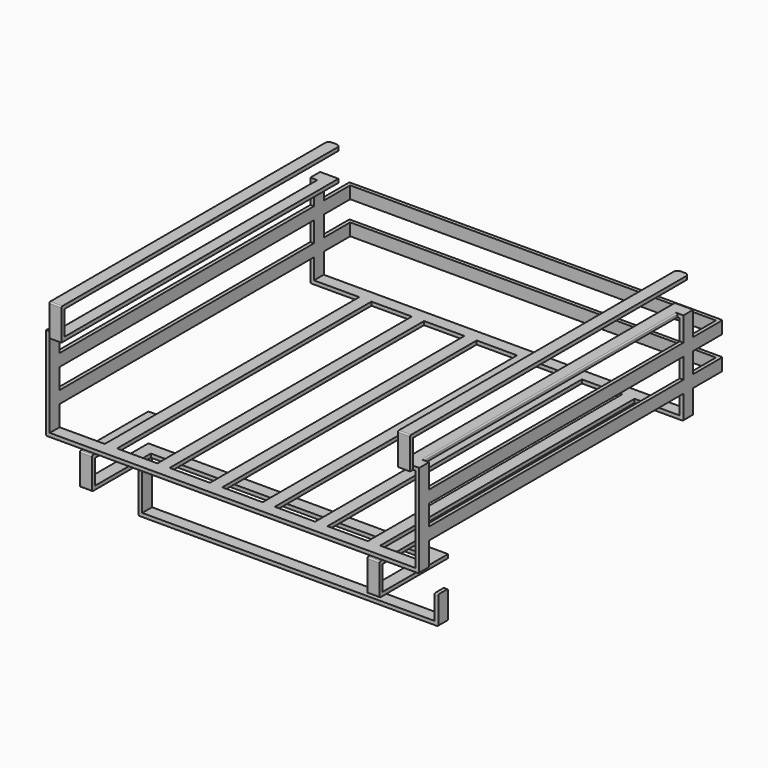
from build123d import *

# Parameters (mm, degrees)
F0_W           = 10
F0_H           = 260
F1_DEPTH       = 3
F2_W           = 3
F2_H           = 10
F3_DEPTH       = 70
F4_W           = 2
F4_H           = 10
F4_W_2         = 3
F4_W_3         = 10
F4_H_2         = 3
F4_W_4         = 5
F5_DEPTH       = 3
F6_W           = 10
F6_H           = 3
F7_DEPTH       = 20
F8_W           = 10
F8_H           = 282
F8_H_2         = 285
F8_H_3         = 3
F9_DEPTH       = 3
F10_W          = 3
F10_H          = 10
F11_DEPTH      = 30
F11_DEPTH_BACK = 270
F12_W          = 3
F12_H          = 10
F13_DEPTH      = 299
F14_R          = 1
F15_R          = 3
F16_W          = 10
F16_H          = 70
F17_DEPTH      = 3
F18_W          = 10
F18_H          = 3
F19_DEPTH      = 20
F20_W          = 10
F20_H          = 70
F21_DEPTH      = 3
F20_H_2        = 67
F20_H_3        = 3
F22_W          = 10
F22_H          = 3
F23_DEPTH      = 225
F24_W          = 3
F24_H          = 10
F25_DEPTH      = 45
F26_W          = 10
F26_H          = 3
F27_DEPTH      = 242
F28_W          = 3
F28_H          = 10
F29_DEPTH      = 20
F30_R          = 1
F32_DEPTH      = 1


with BuildPart() as f1:
    # F0 (on Top) → F1 (new body)
    with BuildSketch(Plane.XY):
        Polygon((135.7191348076, 185.6500792865), (-169.2808651924, 185.6500792865), (-169.2808651924, 175.6500792865), (-129.2808651924, 175.6500792865), (-119.2808651924, 175.6500792865), (-86.2808651924, 175.6500792865), (-76.2808651924, 175.6500792865), (-43.2808651924, 175.6500792865), (-33.2808651924, 175.6500792865), (-0.2808651924, 175.6500792865), (9.7191348076, 175.6500792865), (42.7191348076, 175.6500792865), (52.7191348076, 175.6500792865), (85.7191348076, 175.6500792865), (95.7191348076, 175.6500792865), (135.7191348076, 175.6500792865), align=None)
        with Locations((-124.2808651924, 45.6500792865)):
            Rectangle(F0_W, F0_H)
        with Locations((-81.2808651924, 45.6500792865)):
            Rectangle(F0_W, F0_H)
        with Locations((-38.2808651924, 45.6500792865)):
            Rectangle(F0_W, F0_H)
        with Locations((4.7191348076, 45.6500792865)):
            Rectangle(F0_W, F0_H)
        with Locations((47.7191348076, 45.6500792865)):
            Rectangle(F0_W, F0_H)
        with Locations((90.7191348076, 45.6500792865)):
            Rectangle(F0_W, F0_H)
        Polygon((-129.2808651924, -84.3499207135), (-169.2808651924, -84.3499207135), (-169.2808651924, -94.3499207135), (135.7191348076, -94.3499207135), (135.7191348076, -84.3499207135), (95.7191348076, -84.3499207135), (85.7191348076, -84.3499207135), (52.7191348076, -84.3499207135), (42.7191348076, -84.3499207135), (9.7191348076, -84.3499207135), (-0.2808651924, -84.3499207135), (-33.2808651924, -84.3499207135), (-43.2808651924, -84.3499207135), (-76.2808651924, -84.3499207135), (-86.2808651924, -84.3499207135), (-119.2808651924, -84.3499207135), align=None)
    extrude(amount=F1_DEPTH)

    # F2 (on face) → F3 (join)
    with BuildSketch(Plane.XY.offset(3)):
        with Locations((-167.7808651924, 180.6500792865)):
            Rectangle(F2_W, F2_H)
        with Locations((134.2191348076, 180.6500792865)):
            Rectangle(F2_W, F2_H)
        with Locations((134.2191348076, -89.3499207135)):
            Rectangle(F2_W, F2_H)
        with Locations((-167.7808651924, -89.3499207135)):
            Rectangle(F2_W, F2_H)
    extrude(amount=F3_DEPTH)

    # F4 (on face) → F5 (join)
    with BuildSketch(Plane.XY.offset(73)):
        Polygon((-154.2808651924, 185.6500792865), (-164.2808651924, 185.6500792865), (-164.2808651924, 175.6500792865), (-164.2808651924, -84.3499207135), (-164.2808651924, -94.3499207135), (-154.2808651924, -94.3499207135), align=None)
        with Locations((-165.2808651924, 180.6500792865)):
            Rectangle(F4_W, F4_H)
        with Locations((-167.7808651924, 180.6500792865)):
            Rectangle(F4_W_2, F4_H)
        with Locations((-159.2808651924, -95.8499207135)):
            Rectangle(F4_W_3, F4_H_2)
        with Locations((125.7191348076, -95.8499207135)):
            Rectangle(F4_W_3, F4_H_2)
        Polygon((130.7191348076, 185.6500792865), (120.7191348076, 185.6500792865), (120.7191348076, -94.3499207135), (130.7191348076, -94.3499207135), (130.7191348076, -84.3499207135), (130.7191348076, 175.6500792865), align=None)
        with Locations((133.2191348076, -89.3499207135)):
            Rectangle(F4_W_4, F4_H)
        with Locations((133.2191348076, 180.6500792865)):
            Rectangle(F4_W_4, F4_H)
        with Locations((-166.7808651924, -89.3499207135)):
            Rectangle(F4_W_4, F4_H)
    extrude(amount=F5_DEPTH)

    # F6 (on face) → F7 (join)
    with BuildSketch(Plane.XY.offset(76)):
        with Locations((-159.2808651924, -95.8499207135)):
            Rectangle(F6_W, F6_H)
        with Locations((125.7191348076, -95.8499207135)):
            Rectangle(F6_W, F6_H)
    extrude(amount=F7_DEPTH)

    # F8 (on face) → F9 (join)
    with BuildSketch(Plane.XY.offset(96)):
        with Locations((-159.2808651924, 46.6500792865)):
            Rectangle(F8_W, F8_H)
        with Locations((125.7191348076, 45.1500792865)):
            Rectangle(F8_W, F8_H_2)
        with Locations((-159.2808651924, -95.8499207135)):
            Rectangle(F8_W, F8_H_3)
    extrude(amount=F9_DEPTH)

    # F10 (on face) → F11 (join, two sides)
    with BuildSketch(Plane(origin=(0, 185.6500792865, 0), x_dir=(-1, 0, 0), z_dir=(0, 1, 0))) as f11_sk:
        with Locations((167.7808651924, 51.3333333333)):
            Rectangle(F10_W, F10_H)
        with Locations((167.7808651924, 24.6666666667)):
            Rectangle(F10_W, F10_H)
        with Locations((-134.2191348076, 51.3333333333)):
            Rectangle(F10_W, F10_H)
        with Locations((-134.2191348076, 24.6666666667)):
            Rectangle(F10_W, F10_H)
    extrude(amount=F11_DEPTH)
    extrude(f11_sk.sketch, amount=-F11_DEPTH_BACK)

    # F12 (on face) → F13 (join, through all)
    with BuildSketch(Plane.YZ.offset(-166.2808651924)):
        with Locations((214.1500792864, 51.3333333333)):
            Rectangle(F12_W, F12_H)
        with Locations((214.1500792864, 24.6666666667)):
            Rectangle(F12_W, F12_H)
    extrude(amount=F13_DEPTH)

    # F14
    f14_edges = [f1.edges().sort_by_distance(p)[0] for p in [
        (-169.280865, 180.650079, 0),
        (-169.280865, -89.349921, 0),
        (135.719135, -89.349921, 0),
        (135.719135, 180.650079, 0),
        (135.719135, 215.650079, 24.666667),
        (135.719135, 215.650079, 51.333333),
        (-169.280865, 215.650079, 51.333333),
        (-169.280865, 215.650079, 24.666667),
        (-164.280865, 45.650079, 76),
        (-159.280865, -97.349921, 99),
        (125.719135, -97.349921, 99),
        (130.719135, 45.650079, 76),
    ]]
    fillet(f14_edges, radius=F14_R)

    # F15
    f15_edges = [f1.edges().sort_by_distance(p)[0] for p in [
        (-154.280865, 187.650079, 97.5),
        (-164.280865, 187.650079, 97.5),
        (120.719135, 187.650079, 97.5),
        (130.719135, 187.650079, 97.5),
    ]]
    fillet(f15_edges, radius=F15_R)


with BuildPart() as f17:
    # F16 (on Top) → F17 (new body)
    with BuildSketch(Plane.XY):
        with Locations((-134.2808651924, -62.3499207135)):
            Rectangle(F16_W, F16_H)
    extrude(amount=-F17_DEPTH)

    # F18 (on face) → F19 (join)
    with BuildSketch(Plane(origin=(0, 0, -3), x_dir=(1, 0, 0), z_dir=(0, 0, -1))):
        with Locations((-134.2808651924, 95.8499207135)):
            Rectangle(F18_W, F18_H)
    extrude(amount=F19_DEPTH)

    # F20 (on face) → F21, piece 2 (join)
    with BuildSketch(Plane(origin=(0, 0, -23), x_dir=(1, 0, 0), z_dir=(0, 0, -1))):
        with Locations((-134.2808651924, 60.8499207135)):
            Rectangle(F20_W, F20_H_2)
        with Locations((-134.2808651924, 95.8499207135)):
            Rectangle(F20_W, F20_H_3)
    extrude(amount=F21_DEPTH)



with BuildPart() as f17b:
    # F16 (on Top) → F17, piece 2 (new body)
    with BuildSketch(Plane.XY):
        with Locations((100.7191348076, -62.3499207135)):
            Rectangle(F16_W, F16_H)
    extrude(amount=-F17_DEPTH)

    # F18 (on face) → F19, piece 2 (join)
    with BuildSketch(Plane(origin=(0, 0, -3), x_dir=(1, 0, 0), z_dir=(0, 0, -1))):
        with Locations((100.7191348076, 95.8499207135)):
            Rectangle(F18_W, F18_H)
    extrude(amount=F19_DEPTH)

    # F20 (on face) → F21 (join)
    with BuildSketch(Plane(origin=(0, 0, -23), x_dir=(1, 0, 0), z_dir=(0, 0, -1))):
        with Locations((100.7191348076, 62.3499207135)):
            Rectangle(F20_W, F20_H)
    extrude(amount=F21_DEPTH)


with BuildPart() as f17_1:
    add(f17.part)

    add(f17b.part)  # F23 merges F17b
    # F22 (on face) → F23 (join, through all)
    with BuildSketch(Plane.YZ.offset(-129.2808651924)):
        with Locations((-32.3499207135, -24.5)):
            Rectangle(F22_W, F22_H)
    extrude(amount=F23_DEPTH)

    # F24 (on face) → F25 (join)
    with BuildSketch(Plane(origin=(0, 0, -26), x_dir=(1, 0, 0), z_dir=(0, 0, -1))):
        with Locations((-137.7808651924, 32.3499207135)):
            Rectangle(F24_W, F24_H)
    extrude(amount=F25_DEPTH)

    # F26 (on face) → F27 (join, through all)
    with BuildSketch(Plane.YZ.offset(-136.2808651924)):
        with Locations((-32.3499207135, -69.5)):
            Rectangle(F26_W, F26_H)
    extrude(amount=F27_DEPTH)

    # F28 (on face) → F29 (join)
    with BuildSketch(Plane.XY.offset(-68)):
        with Locations((104.2191348077, -32.3499207135)):
            Rectangle(F28_W, F28_H)
    extrude(amount=F29_DEPTH)

    # F30
    f30_edges = [f17_1.edges().sort_by_distance(p)[0] for p in [
        (-129.280865, -27.349921, -1.5),
        (-139.280865, -27.349921, -1.5),
        (-134.280865, -97.349921, 0),
        (-134.280865, -97.349921, -26),
        (100.719135, -97.349921, 0),
        (100.719135, -97.349921, -26),
        (95.719135, -27.349921, -1.5),
        (105.719135, -27.349921, -1.5),
        (-139.280865, -32.349921, -71),
        (105.719135, -32.349921, -71),
        (104.219135, -37.349921, -48),
        (104.219135, -27.349921, -48),
    ]]
    fillet(f30_edges, radius=F30_R)


with BuildPart() as f32:
    # F31 (on face) → F32 (new body)
    with BuildSketch(Plane(origin=(0, 0, -3), x_dir=(1, 0, 0), z_dir=(0, 0, -1))):
        with BuildLine():
            ThreePointArc((-138.1987937689, 35.725209862), (-134.1987937689, 31.725209862), (-130.1987937689, 35.725209862))
            Line((-130.1987937689, 35.725209862), (-130.1987937689, 52.725209862))
            ThreePointArc((-130.1987937689, 52.725209862), (-134.1987937689, 56.725209862), (-138.1987937689, 52.725209862))
            Line((-138.1987937689, 52.725209862), (-138.1987937689, 35.725209862))
        make_face()
    extrude(amount=F32_DEPTH)


with BuildPart() as f32b:
    # F31 (on face) → F32, piece 2 (new body)
    with BuildSketch(Plane(origin=(0, 0, -3), x_dir=(1, 0, 0), z_dir=(0, 0, -1))):
        with BuildLine():
            ThreePointArc((104.6370633841, 52.725209862), (100.6370633841, 56.725209862), (96.6370633841, 52.725209862))
            Line((96.6370633841, 52.725209862), (96.6370633841, 35.725209862))
            ThreePointArc((96.6370633841, 35.725209862), (100.6370633841, 31.725209862), (104.6370633841, 35.725209862))
            Line((104.6370633841, 35.725209862), (104.6370633841, 52.725209862))
        make_face()
    extrude(amount=F32_DEPTH)


with BuildPart() as f32c:
    # F31 (on face) → F32, piece 3 (new body)
    with BuildSketch(Plane(origin=(0, 0, -3), x_dir=(1, 0, 0), z_dir=(0, 0, -1))):
        with BuildLine():
            ThreePointArc((104.6370633841, 86.9746315651), (100.6370633841, 90.9746315651), (96.6370633841, 86.9746315651))
            Line((96.6370633841, 86.9746315651), (96.6370633841, 69.9746315651))
            ThreePointArc((96.6370633841, 69.9746315651), (100.6370633841, 65.9746315651), (104.6370633841, 69.9746315651))
            Line((104.6370633841, 69.9746315651), (104.6370633841, 86.9746315651))
        make_face()
    extrude(amount=F32_DEPTH)


with BuildPart() as f32d:
    # F31 (on face) → F32, piece 4 (new body)
    with BuildSketch(Plane(origin=(0, 0, -3), x_dir=(1, 0, 0), z_dir=(0, 0, -1))):
        with BuildLine():
            Line((-138.1987937689, 86.9746315651), (-138.1987937689, 69.9746315651))
            ThreePointArc((-138.1987937689, 69.9746315651), (-134.1987937689, 65.9746315651), (-130.1987937689, 69.9746315651))
            Line((-130.1987937689, 69.9746315651), (-130.1987937689, 86.9746315651))
            ThreePointArc((-130.1987937689, 86.9746315651), (-134.1987937689, 90.9746315651), (-138.1987937689, 86.9746315651))
        make_face()
    extrude(amount=F32_DEPTH)


solid = Compound([f1.part, f17_1.part, f32.part, f32b.part, f32c.part, f32d.part])
